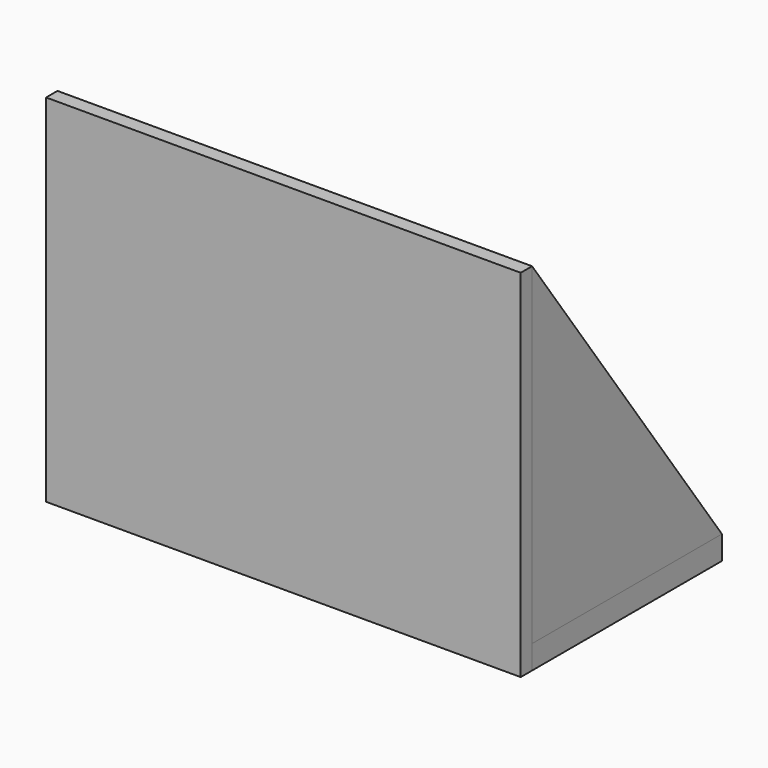
from build123d import *

# Parameters (mm, degrees)
F0_W     = 100
F0_H     = 50
F1_DEPTH = 2.5
F2_W     = 100
F2_H     = 70
F2_H_2   = 5
F3_DEPTH = 3
F5_DEPTH = 5
F8_D     = 7


with BuildPart() as f1:
    # F0 (on Top) → F1 (new body, symmetric)
    with BuildSketch(Plane.XY):
        Rectangle(F0_W, F0_H)
    extrude(amount=F1_DEPTH, both=True)

    # F8 (through all)
    with Locations(Plane.XY.offset(2.5)):
        with Locations((-20, -10), (20, -10), (-20, 10), (20, 10)):
            Hole(F8_D / 2)


with BuildPart() as f3:
    # F2 (on face) → F3 (new body)
    with BuildSketch(Plane.XZ.offset(25)):
        with Locations((0, 37.5)):
            Rectangle(F2_W, F2_H)
        Rectangle(F2_W, F2_H_2)
    extrude(amount=F3_DEPTH)


with BuildPart() as f5:
    # F4 (on face) → F5 (new body)
    with BuildSketch(Plane.YZ.offset(50)):
        Polygon((25, 2.5), (-25, 72.5), (-25, 2.5), align=None)
    extrude(amount=-F5_DEPTH)


with BuildPart() as f6_1:
    # F6: instance of F5
    add(f5.part.mirror(Plane.YZ))


solid = Compound([f1.part, f3.part, f5.part, f6_1.part])
